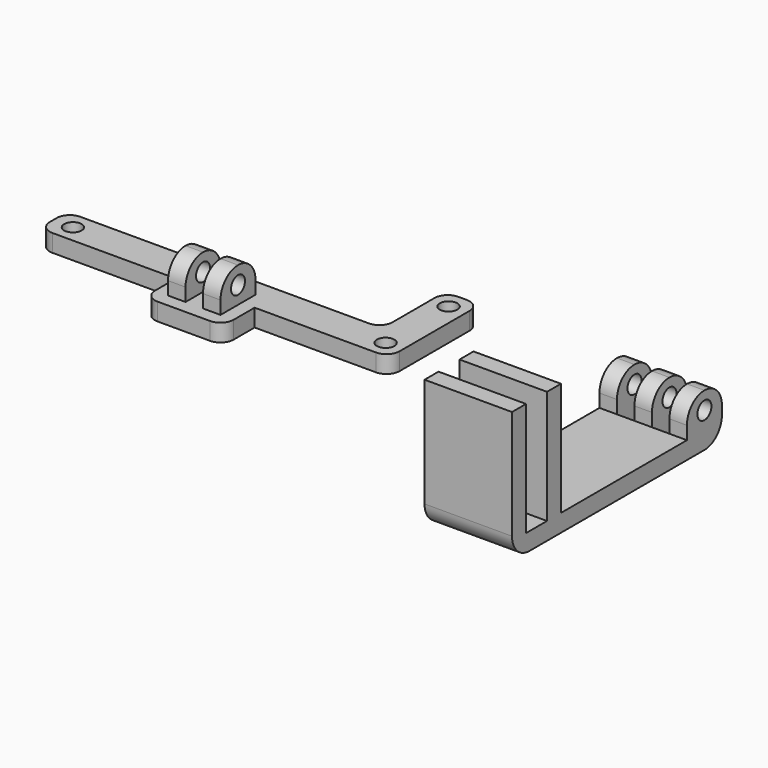
from build123d import *

# Parameters (mm, degrees)
F0_W      = 80
F0_H      = 35
F1_DEPTH  = 4
F2_R      = 2
F2_W      = 78.2012213022
F2_H      = 24.0091495216
F3_DEPTH  = 25
F4_W      = 4
F4_H      = 10
F5_DEPTH  = 8
F6_R      = 2
F7_DEPTH  = 12
F8_R      = 4.99999
F9_W      = 30.75
F9_H      = 9
F9_W_2    = 31.25
F10_DEPTH = 25
F11_R     = 3
F12_W     = 20
F12_H     = 60
F13_DEPTH = 4
F14_W     = 10
F14_H     = 8
F14_W_2   = 14
F14_H_2   = 26
F15_DEPTH = 20
F16_R     = 2
F16_W     = 6
F16_H     = 26
F17_DEPTH = 20
F18_W     = 4
F18_H     = 10
F19_DEPTH = 12
F20_R     = 4.99999


# Not quite as in the source:
# - a fillet or chamfer is up to 0.001 mm smaller than in the source, because OpenCascade refuses the exact size


with BuildPart() as f1:
    # F0 (on Top) → F1 (new body)
    with BuildSketch(Plane.XY):
        with Locations((-49.6926223859, 45.5681574084)):
            Rectangle(F0_W, F0_H)
    extrude(amount=F1_DEPTH)

    # F2 (on face) → F3 (cut)
    with BuildSketch(Plane.XY.offset(4)):
        with Locations((-85.1926223859, 41.0681574084)):
            Circle(F2_R)
        with Locations((-13.6926223859, 41.0681574084)):
            Circle(F2_R)
        with Locations((-13.6926223859, 59.0681574084)):
            Circle(F2_R)
        with Locations((-56.793233037, 57.0727321692)):
            Rectangle(F2_W, F2_H)
    extrude(amount=-F3_DEPTH, mode=Mode.SUBTRACT)

    # F4 (on face) → F5 (join)
    with BuildSketch(Plane.XY.offset(4)):
        with Locations((-53.4426223859, 36.0681574084)):
            Rectangle(F4_W, F4_H)
        with Locations((-45.4426223859, 36.0681574084)):
            Rectangle(F4_W, F4_H)
    extrude(amount=F5_DEPTH)

    # F6 (on face) → F7 (cut)
    with BuildSketch(Plane(origin=(-55.4426223859, 0, 0), x_dir=(0, -1, 0), z_dir=(-1, 0, 0))):
        with Locations((-36.0681574084, 8)):
            Circle(F6_R)
    extrude(amount=-F7_DEPTH, mode=Mode.SUBTRACT)

    # F8 (radius 5 in the source; OpenCascade refuses exactly that, so slightly less here)
    f8_edges = [f1.edges().sort_by_distance(p)[0] for p in [
        (-53.442622, 41.068157, 12),
        (-45.442622, 41.068157, 12),
        (-53.442622, 31.068157, 12),
        (-45.442622, 31.068157, 12),
    ]]
    fillet(f8_edges, radius=F8_R)

    # F9 (on face) → F10 (cut)
    with BuildSketch(Plane.XY.offset(4)):
        Polygon((-89.6926223859, 37.0681574084), (-102.8804979962, 37.0681574084), (-102.8804979962, 18.9452479413), (-58.4426223859, 18.9452479413), (-58.4426223859, 28.0681574084), (-89.6926223859, 28.0681574084), align=None)
        Polygon((-9.6926223859, 28.0681574084), (-40.4426223859, 28.0681574084), (-40.4426223859, 16.9630516109), (3.4488050875, 16.9630516109), (3.4488050875, 37.0681574084), (-9.6926223859, 37.0681574084), align=None)
        with Locations((-25.0676223859, 32.5681574084)):
            Rectangle(F9_W, F9_H)
        with Locations((-74.0676223859, 32.5681574084)):
            Rectangle(F9_W_2, F9_H)
    extrude(amount=-F10_DEPTH, mode=Mode.SUBTRACT)

    # F11
    f11_edges = [f1.edges().sort_by_distance(p)[0] for p in [
        (-89.692622, 45.068157, 2),
        (-89.692622, 37.068157, 2),
        (-58.442622, 28.068157, 2),
        (-40.442622, 28.068157, 2),
        (-9.692622, 37.068157, 2),
        (-9.692622, 63.068157, 2),
        (-17.692622, 63.068157, 2),
        (-17.692622, 45.068157, 2),
    ]]
    fillet(f11_edges, radius=F11_R)


with BuildPart() as f13:
    # F12 (on Top) → F13 (new body)
    with BuildSketch(Plane.XY):
        with Locations((41.8533885479, 25.26676815)):
            Rectangle(F12_W, F12_H)
    extrude(amount=F13_DEPTH)

    # F14 (on face) → F15 (join)
    with BuildSketch(Plane.YZ.offset(51.8533885479)):
        with Locations((50.26676815, 8)):
            Rectangle(F14_W, F14_H)
        with Locations((2.26676815, 17)):
            Rectangle(F14_W_2, F14_H_2)
    extrude(amount=-F15_DEPTH)

    # F16 (on face) → F17 (cut)
    with BuildSketch(Plane.YZ.offset(51.8533885479)):
        with Locations((50.26676815, 8)):
            Circle(F16_R)
        with Locations((2.26676815, 17)):
            Rectangle(F16_W, F16_H)
    extrude(amount=-F17_DEPTH, mode=Mode.SUBTRACT)

    # F18 (on face) → F19 (cut)
    with BuildSketch(Plane.XY.offset(12)):
        with Locations((37.8533885479, 50.26676815)):
            Rectangle(F18_W, F18_H)
        with Locations((45.8533885479, 50.26676815)):
            Rectangle(F18_W, F18_H)
    extrude(amount=-F19_DEPTH, mode=Mode.SUBTRACT)

    # F20 (radius 5 in the source; OpenCascade refuses exactly that, so slightly less here)
    f20_edges = [f13.edges().sort_by_distance(p)[0] for p in [
        (41.853389, -4.733232, 0),
        (49.853389, 45.266768, 12),
        (49.853389, 55.266768, 12),
        (41.853389, 45.266768, 12),
        (41.853389, 55.266768, 12),
        (33.853389, 45.266768, 12),
        (33.853389, 55.266768, 12),
        (49.853389, 55.266768, 0),
        (41.853389, 55.266768, 0),
        (33.853389, 55.266768, 0),
    ]]
    fillet(f20_edges, radius=F20_R)


solid = Compound([f1.part, f13.part])
